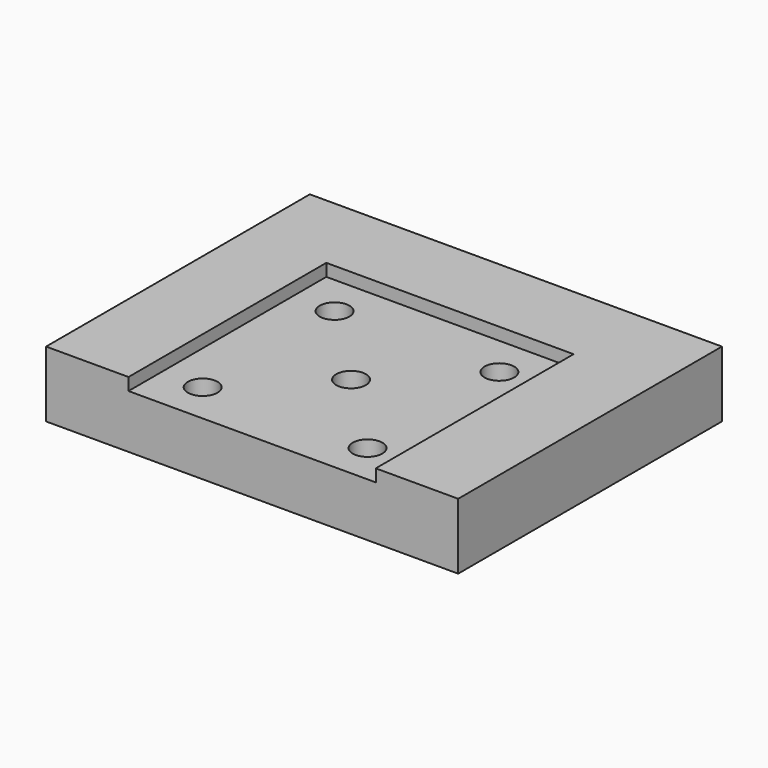
from build123d import *
from build123d import SkipClean  # not in build123d's __all__

# Parameters (mm, degrees)
F0_R      = 2.85
F0_R_2    = 11
F1_DEPTH  = 40
F2_W      = 30
F2_H      = 30
F3_DEPTH  = 55
F5_DEPTH  = 30
F6_DEPTH  = 40.001
F7_DEPTH  = 40.001
F8_R      = 1.8
F9_DEPTH  = 11.5
F10_DEPTH = 13
F11_DEPTH = 5


with BuildPart() as f1:
    # F0 (on Front) → F1 (new body)
    with BuildSketch(Plane.XZ):
        with BuildLine():
            Line((15, 28.25), (-15, 28.25))
            ThreePointArc((-15, 28.25), (-22.0710678119, 25.3210678119), (-25, 18.25))
            Line((-25, 18.25), (-25, -38.25))
            Line((-25, -38.25), (25, -38.25))
            Line((25, -38.25), (25, 18.25))
            ThreePointArc((25, 18.25), (22.0710678119, 25.3210678119), (15, 28.25))
        make_face()
        with Locations((0, -18.25)):
            Circle(F0_R, mode=Mode.SUBTRACT)
        Circle(F0_R_2, mode=Mode.SUBTRACT)
        with Locations((0, 18.25)):
            Circle(F0_R, mode=Mode.SUBTRACT)
    extrude(amount=F1_DEPTH)

    # F2 (on face) → F3 (cut)
    with BuildSketch(Plane.XY.offset(28.25)):
        with Locations((0, -25)):
            Rectangle(F2_W, F2_H)
    extrude(amount=-F3_DEPTH, mode=Mode.SUBTRACT)

    # F4 (on face) → F5 (join, through all)
    with BuildSketch(Plane.XZ.offset(40)):
        with BuildLine():
            Line((-15, 17.2291616466), (-15, 19.972135955))
            ThreePointArc((-15, 19.972135955), (-20, 15.5), (-15, 11.027864045))
            Line((-15, 11.027864045), (-15, 13.7708383534))
            ThreePointArc((-15, 13.7708383534), (-17.3, 15.5), (-15, 17.2291616466))
        make_face()
        with BuildLine():
            Line((-15, -17.2291616466), (-15, -19.972135955))
            ThreePointArc((-15, -19.972135955), (-12.1458980338, -18.5), (-11, -15.5))
            ThreePointArc((-11, -15.5), (-12.1458980338, -12.5), (-15, -11.027864045))
            Line((-15, -11.027864045), (-15, -13.7708383534))
            ThreePointArc((-15, -13.7708383534), (-14.061250543, -14.4183346174), (-13.7, -15.5))
            ThreePointArc((-13.7, -15.5), (-14.061250543, -16.5816653826), (-15, -17.2291616466))
        make_face()
        with BuildLine():
            ThreePointArc((20, -15.5), (18.5, -12.1458980338), (15, -11.027864045))
            Line((15, -11.027864045), (15, -13.7708383534))
            ThreePointArc((15, -13.7708383534), (16.5816653826, -14.061250543), (17.3, -15.5))
            ThreePointArc((17.3, -15.5), (16.5816653826, -16.938749457), (15, -17.2291616466))
            Line((15, -17.2291616466), (15, -19.972135955))
            ThreePointArc((15, -19.972135955), (18.5, -18.8541019662), (20, -15.5))
        make_face()
        with BuildLine():
            Line((15, 17.2291616466), (15, 19.972135955))
            ThreePointArc((15, 19.972135955), (11, 15.5), (15, 11.027864045))
            Line((15, 11.027864045), (15, 13.7708383534))
            ThreePointArc((15, 13.7708383534), (13.7, 15.5), (15, 17.2291616466))
        make_face()
    extrude(amount=-F5_DEPTH)

    # F4 (on face) → F6 (cut, through all)
    with BuildSketch(Plane.XZ.offset(40)):
        with BuildLine():
            ThreePointArc((-13.7, 15.5), (-14.061250543, 16.5816653826), (-15, 17.2291616466))
            Line((-15, 17.2291616466), (-15, 13.7708383534))
            ThreePointArc((-15, 13.7708383534), (-14.061250543, 14.4183346174), (-13.7, 15.5))
        make_face()
        with BuildLine():
            ThreePointArc((17.3, 15.5), (16.5816653826, 16.938749457), (15, 17.2291616466))
            Line((15, 17.2291616466), (15, 13.7708383534))
            ThreePointArc((15, 13.7708383534), (16.5816653826, 14.061250543), (17.3, 15.5))
        make_face()
        with BuildLine():
            Line((15, -17.2291616466), (15, -13.7708383534))
            ThreePointArc((15, -13.7708383534), (13.7, -15.5), (15, -17.2291616466))
        make_face()
        with BuildLine():
            ThreePointArc((-15, -13.7708383534), (-17.3, -15.5), (-15, -17.2291616466))
            Line((-15, -17.2291616466), (-15, -13.7708383534))
        make_face()
    with SkipClean():  # cleaning this boolean's faces spoils the solid; the shape is the same uncleaned
        extrude(amount=-F6_DEPTH, mode=Mode.SUBTRACT)

    # F4 (on face) → F7 (cut, through all)
    with BuildSketch(Plane.XZ.offset(40)):
        with BuildLine():
            Line((-15, 13.7708383534), (-15, 17.2291616466))
            ThreePointArc((-15, 17.2291616466), (-17.3, 15.5), (-15, 13.7708383534))
        make_face()
        with BuildLine():
            Line((15, 13.7708383534), (15, 17.2291616466))
            ThreePointArc((15, 17.2291616466), (13.7, 15.5), (15, 13.7708383534))
        make_face()
        with BuildLine():
            Line((-15, -13.7708383534), (-15, -17.2291616466))
            ThreePointArc((-15, -17.2291616466), (-14.061250543, -16.5816653826), (-13.7, -15.5))
            ThreePointArc((-13.7, -15.5), (-14.061250543, -14.4183346174), (-15, -13.7708383534))
        make_face()
        with BuildLine():
            ThreePointArc((17.3, -15.5), (16.5816653826, -14.061250543), (15, -13.7708383534))
            Line((15, -13.7708383534), (15, -17.2291616466))
            ThreePointArc((15, -17.2291616466), (16.5816653826, -16.938749457), (17.3, -15.5))
        make_face()
    with SkipClean():  # cleaning this boolean's faces spoils the solid; the shape is the same uncleaned
        extrude(amount=-F7_DEPTH, mode=Mode.SUBTRACT)

    # F8 (on face) → F9 (cut, through all)
    with BuildSketch(Plane.XY.offset(-26.75)):
        with Locations((-10, -15)):
            Circle(F8_R)
        with Locations((10, -15)):
            Circle(F8_R)
        with Locations((-10, -35)):
            Circle(F8_R)
        with Locations((10, -35)):
            Circle(F8_R)
        with Locations((0, -25)):
            Circle(F8_R)
    extrude(amount=-F9_DEPTH, mode=Mode.SUBTRACT)

    # F10 (intersect): a face of the model
    f10_faces = [f1.faces().sort_by_distance(p)[0] for p in [
        (0, -19.8694432325, -38.25),
    ]]
    extrude(f10_faces, amount=-F10_DEPTH, mode=Mode.INTERSECT)

    # F11 (cut): a face of the model
    f11_faces = [f1.faces().sort_by_distance(p)[0] for p in [
        (0, -19.8694432325, -38.25),
    ]]
    extrude(f11_faces, amount=-F11_DEPTH, mode=Mode.SUBTRACT)


solid = f1.part
